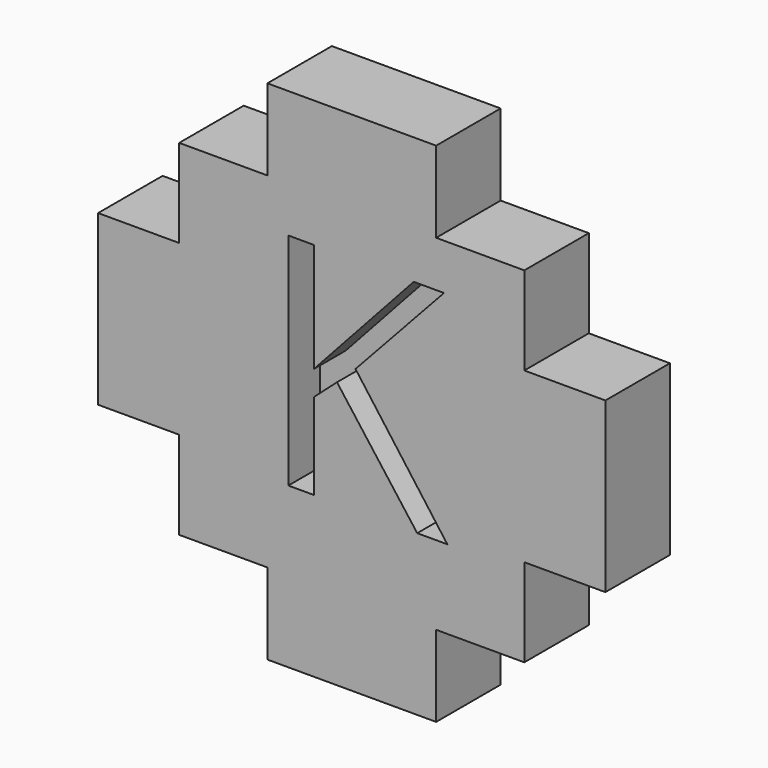
from build123d import *

# Parameters (mm, degrees)
F1_DEPTH     = 2.032
F2_TEXT_SIZE = 7.7734513889
F3_DEPTH     = 1


# Not quite as in the source:
# - a length typed as a fraction of an inch, garbled in the dataset ("3 / 203.2 mm" for 3/8 in), is restored
# - Text() gives the source's letters only with a copy of the font that has no kerning and outlines rounded to 1/6400 em; it was checked with that copy


with BuildPart() as f1:
    # F0 (on Front) → F1 (new body)
    with BuildSketch(Plane.XZ):
        Polygon((-15.2212520439, 36.2265945869), (-17.3485020439, 36.2265945869), (-19.4757520439, 36.2265945869), (-19.4757520439, 34.1818945869), (-21.6982520439, 34.1818945869), (-21.6982520439, 31.9593945869), (-23.7429520439, 31.9593945869), (-23.7429520439, 29.8321445869), (-23.7429520439, 27.7048945869), (-21.6982520439, 27.7048945869), (-21.6982520439, 25.4823945869), (-19.4757520439, 25.4823945869), (-19.4757520439, 23.4376945869), (-17.3485020439, 23.4376945869), (-15.2212520439, 23.4376945869), (-15.2212520439, 25.4823945869), (-12.9987520439, 25.4823945869), (-12.9987520439, 27.7048945869), (-10.9540520439, 27.7048945869), (-10.9540520439, 29.8321445869), (-10.9540520439, 31.9593945869), (-12.9987520439, 31.9593945869), (-12.9987520439, 34.1818945869), (-15.2212520439, 34.1818945869), align=None)
    extrude(amount=F1_DEPTH)

    # F2 (on face) → F3 (cut)
    with BuildSketch(Plane.XZ.offset(2.032)):
        with Locations((-19.709998706, 27.4716445021)):
            Text('K', F2_TEXT_SIZE, font='Open Sans', text_align=(TextAlign.LEFT, TextAlign.BOTTOM))
    extrude(amount=-F3_DEPTH, mode=Mode.SUBTRACT)


solid = f1.part
